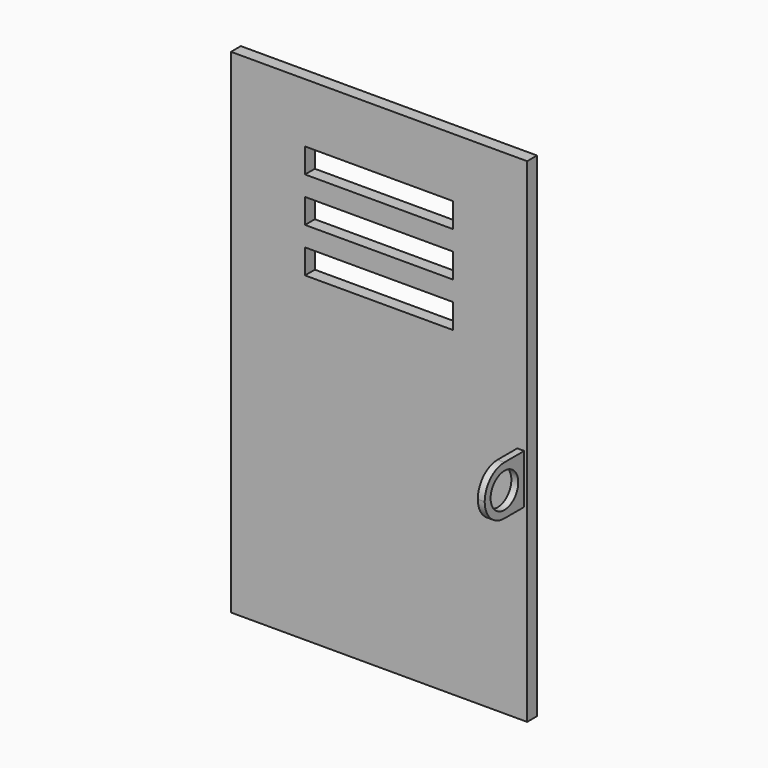
from build123d import *

# Parameters (mm, degrees)
F0_W     = 76.2
F0_H     = 127
F1_DEPTH = 3.175
F2_W     = 38.1
F2_H     = 6.35
F3_DEPTH = 3.175
F4_W     = 1.778
F4_H     = 12.7
F5_DEPTH = 12.7
F6_R     = 6.35
F7_R     = 6.34999
F8_R     = 4.445
F9_DEPTH = 25.4


# Not quite as in the source:
# - a fillet or chamfer is up to 0.001 mm smaller than in the source, because OpenCascade refuses the exact size


with BuildPart() as f1:
    # F0 (on Front) → F1 (new body)
    with BuildSketch(Plane.XZ):
        with Locations((1.208204776, 15.0653144508)):
            Rectangle(F0_W, F0_H)
    extrude(amount=F1_DEPTH)

    # F2 (on face) → F3 (cut)
    with BuildSketch(Plane.XZ.offset(3.175)):
        with Locations((1.208204776, 60.1503144508)):
            Rectangle(F2_W, F2_H)
        with Locations((1.208204776, 48.7203144508)):
            Rectangle(F2_W, F2_H)
        with Locations((1.208204776, 37.2903144508)):
            Rectangle(F2_W, F2_H)
    extrude(amount=-F3_DEPTH, mode=Mode.SUBTRACT)

    # F4 (on face) → F5 (join)
    with BuildSketch(Plane.XZ.offset(3.175)):
        with Locations((37.657204776, 6.35)):
            Rectangle(F4_W, F4_H)
    extrude(amount=F5_DEPTH)

    # F6
    f6_edges = [f1.edges().sort_by_distance(p)[0] for p in [
        (37.657205, -15.875, 12.7),
    ]]
    fillet(f6_edges, radius=F6_R)

    # F7 (radius 6.35 in the source; OpenCascade refuses exactly that, so slightly less here)
    f7_edges = [f1.edges().sort_by_distance(p)[0] for p in [
        (37.657205, -15.875, 0),
    ]]
    fillet(f7_edges, radius=F7_R)

    # F8 (on face) → F9 (cut)
    with BuildSketch(Plane(origin=(36.768204776, 0, 0), x_dir=(0, -1, 0), z_dir=(-1, 0, 0))):
        with Locations((9.525, 6.35)):
            Circle(F8_R)
    extrude(amount=-F9_DEPTH, mode=Mode.SUBTRACT)


solid = f1.part
